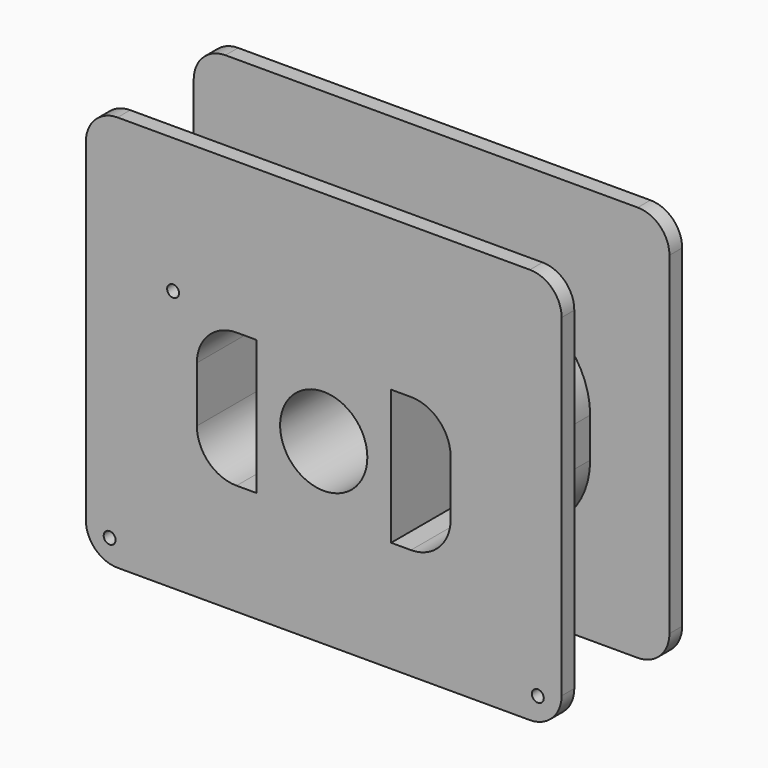
from build123d import *

# Parameters (mm, degrees)
F0_W      = 60
F0_H      = 50
F0_R      = 5.5
F1_DEPTH  = 2
F2_W      = 40
F2_H      = 25
F2_R      = 5.5
F3_DEPTH  = 15
F4_R      = 10
F5_W      = 60
F5_H      = 50
F5_R      = 5.5
F6_DEPTH  = 2
F7_R      = 4
F9_D      = 1.5
F9_DEPTH  = 3
F9_TIP    = 0.4506454643
F10_W     = 7.5
F10_H     = 17
F11_DEPTH = 25
F12_R     = 5


# Not quite as in the source:
# - a feature names something its author has since deleted; it is built from what else it names


with BuildPart() as f1:
    # F0 (on Front) → F1 (new body)
    with BuildSketch(Plane.XZ):
        with Locations((0, 2.5)):
            Rectangle(F0_W, F0_H)
        Circle(F0_R, mode=Mode.SUBTRACT)
    extrude(amount=F1_DEPTH)

    # F2 (on face) → F3 (join)
    with BuildSketch(Plane.XZ.offset(2)):
        Rectangle(F2_W, F2_H)
        Circle(F2_R, mode=Mode.SUBTRACT)
    extrude(amount=F3_DEPTH)

    # F4
    f4_edges = [f1.edges().sort_by_distance(p)[0] for p in [
        (20, -9.5, 12.5),
        (20, -9.5, -12.5),
        (-20, -9.5, -12.5),
        (-20, -9.5, 12.5),
    ]]
    fillet(f4_edges, radius=F4_R)

    # F5 (on face) → F6 (join)
    with BuildSketch(Plane.XZ.offset(17)):
        with Locations((0, 2.5)):
            Rectangle(F5_W, F5_H)
        Circle(F5_R, mode=Mode.SUBTRACT)
    extrude(amount=F6_DEPTH)

    # F7
    f7_edges = [f1.edges().sort_by_distance(p)[0] for p in [
        (30, -18, 27.5),
        (30, -1, 27.5),
        (30, -18, -22.5),
        (30, -1, -22.5),
        (-30, -18, -22.5),
        (-30, -1, -22.5),
        (-30, -18, 27.5),
        (-30, -1, 27.5),
    ]]
    fillet(f7_edges, radius=F7_R)

    # F9
    with Locations(Plane.XZ.offset(19)):
        with Locations((-19, 10.5), (-27, -19.5), (27, -19.5)):
            Hole(F9_D / 2, depth=F9_DEPTH)
            with Locations((0, 0, -(F9_DEPTH + F9_TIP / 2))):  # 118° drill point
                Cone(0, F9_D / 2, F9_TIP, mode=Mode.SUBTRACT)

    # F10 (on face) → F11 (cut)
    with BuildSketch(Plane.XZ.offset(19)):
        with Locations((-12.25, 0)):
            Rectangle(F10_W, F10_H)
        with Locations((12.25, 0)):
            Rectangle(F10_W, F10_H)
    extrude(amount=-F11_DEPTH, mode=Mode.SUBTRACT)

    # F12
    f12_edges = [f1.edges().sort_by_distance(p)[0] for p in [
        (16, -9.5, -8.5),
        (16, -9.5, 8.5),
        (-16, -9.5, 8.5),
        (-16, -9.5, -8.5),
    ]]
    fillet(f12_edges, radius=F12_R)


solid = f1.part
